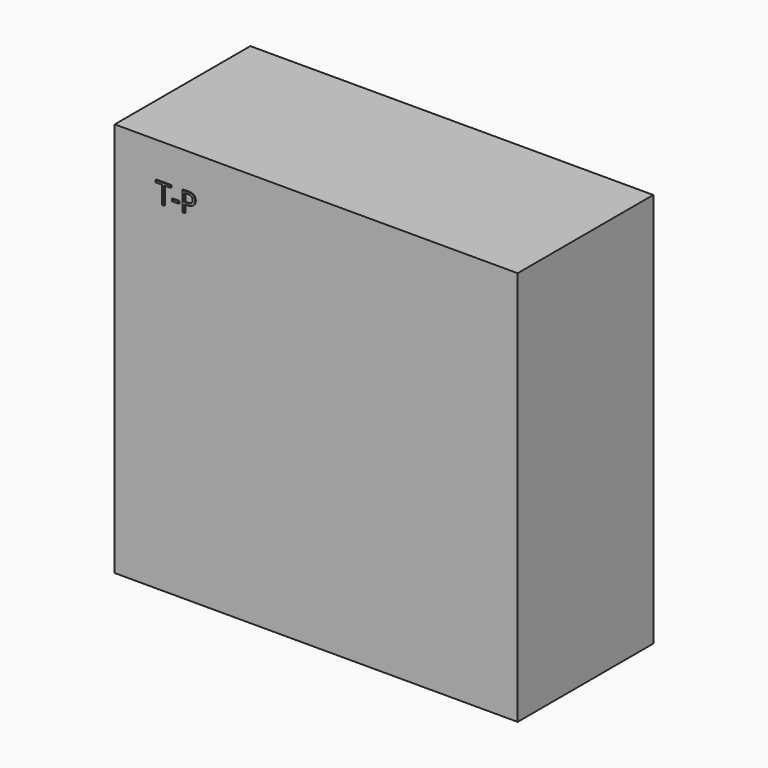
from build123d import *

# Parameters (mm, degrees)
F0_W         = 2422.525
F0_H         = 1019.175
F1_DEPTH     = 2374.9
F2_TEXT_SIZE = 166.8198241128
F3_DEPTH     = 6.35


# Not quite as in the source:
# - Text() gives the source's letters only with a copy of the font that has no kerning and outlines rounded to 1/6400 em; it was checked with that copy


with BuildPart() as f1:
    # F0 (on Top) → F1 (new body)
    with BuildSketch(Plane.XY):
        with Locations((1211.2625, 509.5875)):
            Rectangle(F0_W, F0_H)
    extrude(amount=F1_DEPTH)

    # F2 (on face) → F3 (join)
    with BuildSketch(Plane.XZ):
        with Locations((249.5781928301, 2045.5620288849)):
            Text('T-P', F2_TEXT_SIZE, font='Open Sans', text_align=(TextAlign.LEFT, TextAlign.BOTTOM))
    extrude(amount=F3_DEPTH)


solid = f1.part
